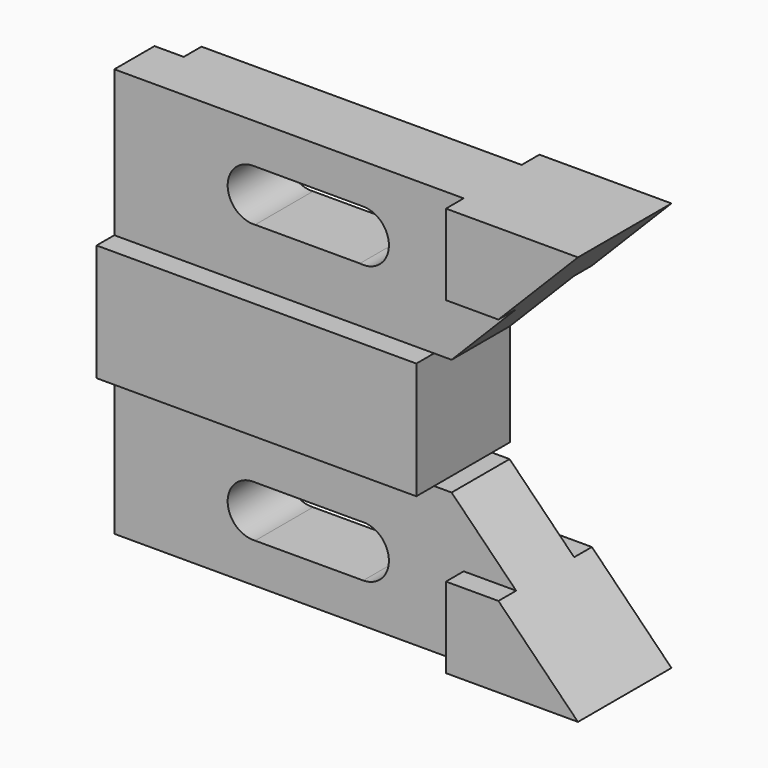
from build123d import *

# Parameters (mm, degrees)
F1_DEPTH      = 12.7
F2_DEPTH      = 7.874
F0_W          = 6.35
F0_H          = 31.75
F3_DEPTH      = 7.874
F3_DEPTH_BACK = 3.048


with BuildPart() as f1:
    # F0 (on Front) → F1 (new body, symmetric)
    with BuildSketch(Plane.XZ):
        Polygon((-54.1707432052, 12.7), (-60.5207432052, 12.7), (-60.5207432052, 0), (8.9898571843, 0), (8.9898571843, 12.7), align=None)
    extrude(amount=F1_DEPTH, both=True)



with BuildPart() as f1b:
    # F0 (on Front) → F1, piece 2 (new body, symmetric)
    with BuildSketch(Plane.XZ):
        Polygon((44.1272567948, 44.45), (15.4252567948, 44.45), (15.4252567948, 26.924), (26.8345322098, 26.924), align=None)
    extrude(amount=F1_DEPTH, both=True)

    # F0 (on Front) → F2 (join, symmetric)
    with BuildSketch(Plane.XZ):
        Polygon((15.4252567948, 44.45), (-54.1707432052, 44.45), (-54.1707432052, 12.7), (8.9898571843, 12.7), (12.7998571843, 12.7), (26.8345322098, 26.924), (15.4252567948, 26.924), align=None)
        with BuildLine():
            ThreePointArc((-29.9125999436, 24.6510820161), (-35.8827432052, 30.226), (-29.9125999436, 35.8009179839))
            Line((-29.9125999436, 35.8009179839), (-6.4141126637, 35.7813519105))
            ThreePointArc((-6.4141126637, 35.7813519105), (-0.8423585797, 29.8335906051), (-7.1321847174, 24.6510820161))
            Line((-7.1321847174, 24.6510820161), (-29.9125999436, 24.6510820161))
        make_face(mode=Mode.SUBTRACT)
    extrude(amount=F2_DEPTH, both=True)

    # F0 (on Front) → F3 (join, two sides)
    with BuildSketch(Plane.XZ) as f3_sk:
        with Locations((-57.3457432052, 28.575)):
            Rectangle(F0_W, F0_H)
    extrude(amount=F3_DEPTH)
    extrude(f3_sk.sketch, amount=-F3_DEPTH_BACK)


with BuildPart() as f1_1:
    add(f1.part)
    # F4: F1b, F1 across plane
    add(f1b.part.mirror(Plane.XY))
    add(f1.part.mirror(Plane.XY))


solid = Compound([f1b.part, f1_1.part])
